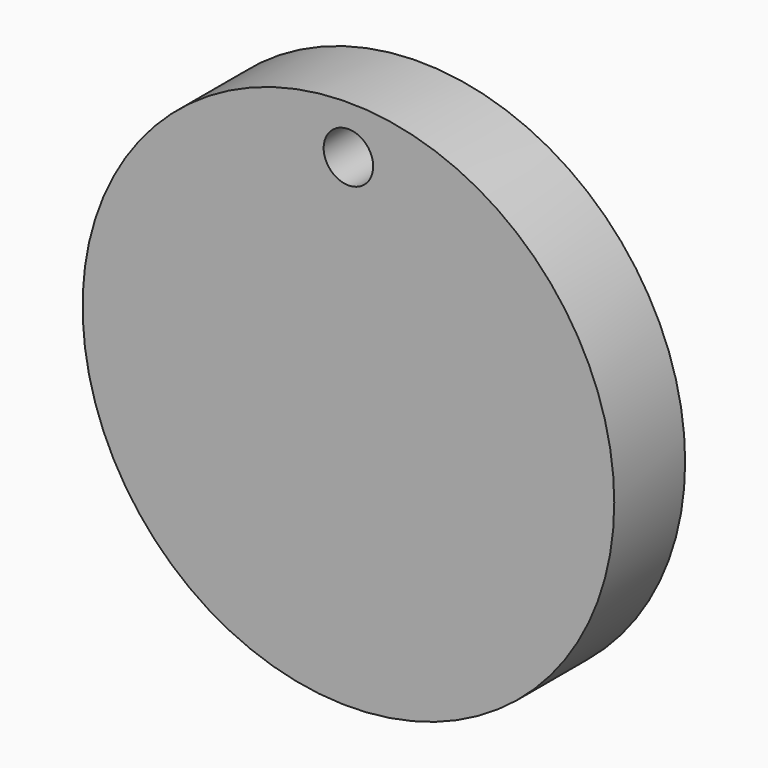
from build123d import *

# Parameters (mm, degrees)
F0_R     = 15
F1_DEPTH = 5
F2_R     = 1.3978994536
F3_DEPTH = 5


# Not quite as in the source:
# - a feature names something its author has since deleted; it is built from what else it names


with BuildPart() as f1:
    # F0 (on Front) → F1 (new body)
    with BuildSketch(Plane.XZ):
        Circle(F0_R)
    extrude(amount=F1_DEPTH)

    # F2 (on face) → F3 (cut)
    with BuildSketch(Plane.XZ.offset(5)):
        with Locations((0, 12.279602699)):
            Circle(F2_R)
    extrude(amount=-F3_DEPTH, mode=Mode.SUBTRACT)


solid = f1.part
